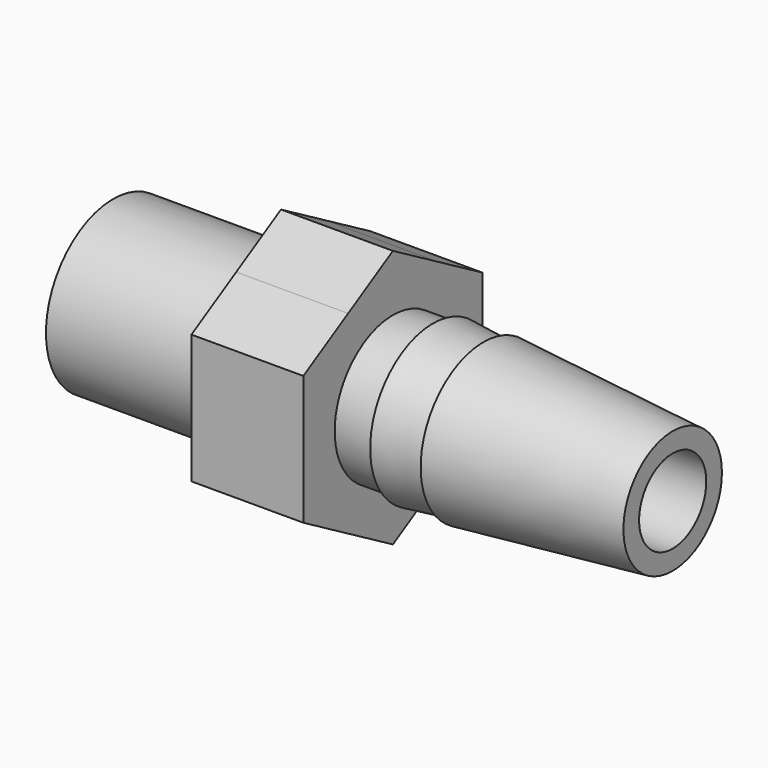
from build123d import *

# Parameters (mm, degrees)
F3_DEPTH = 2


with BuildPart() as f1:
    # F0 (on Top) → F1 (revolve)
    with BuildSketch(Plane.XY):
        Polygon((0, 1.5), (0, 0.75), (10, 0.75), (10, 1.1), (6.6163264594, 1.4), (6.6163264594, 1.3), (5.7138770835, 1.4), (5.7138770835, 1.3), (5, 1.3), (5, 2), (3, 2), (3, 1.5), align=None)
    revolve(axis=Axis((7.7490479817, 0, 0), (1, 0, 0)))

    # F2 (on face) → F3 (join)
    with BuildSketch(Plane.YZ.offset(5)):
        with BuildLine():
            Line((2, 0), (2, 1.1547005384))
            Line((2, 1.1547005384), (1.0000000433, 1.7320507826))
            ThreePointArc((1.0000000433, 1.7320507826), (1.7320508201, 0.9999999783), (2, 0))
        make_face()
        with BuildLine():
            Line((2, -1.1547005384), (2, 0))
            ThreePointArc((2, 0), (1.7320508201, -0.9999999783), (1.0000000433, -1.7320507826))
            Line((1.0000000433, -1.7320507826), (2, -1.1547005384))
        make_face()
        with BuildLine():
            ThreePointArc((-1.0000000602, 1.7320507728), (-9.7e-09, 2), (1.0000000433, 1.7320507826))
            Line((1.0000000433, 1.7320507826), (0, 2.3094010768))
            Line((0, 2.3094010768), (-1.0000000602, 1.7320507728))
        make_face()
        with BuildLine():
            Line((0, -2.3094010768), (1.0000000433, -1.7320507826))
            ThreePointArc((1.0000000433, -1.7320507826), (0, -2), (-1.0000000433, -1.7320507826))
            Line((-1.0000000433, -1.7320507826), (0, -2.3094010768))
        make_face()
        with BuildLine():
            ThreePointArc((-2, 0), (-1.7320508249, 0.9999999699), (-1.0000000602, 1.7320507728))
            Line((-1.0000000602, 1.7320507728), (-2, 1.1547005384))
            Line((-2, 1.1547005384), (-2, 0))
        make_face()
        with BuildLine():
            Line((-2, -1.1547005384), (-1.0000000433, -1.7320507826))
            ThreePointArc((-1.0000000433, -1.7320507826), (-1.7320508201, -0.9999999783), (-2, 0))
            Line((-2, 0), (-2, -1.1547005384))
        make_face()
    extrude(amount=-F3_DEPTH)


solid = f1.part
